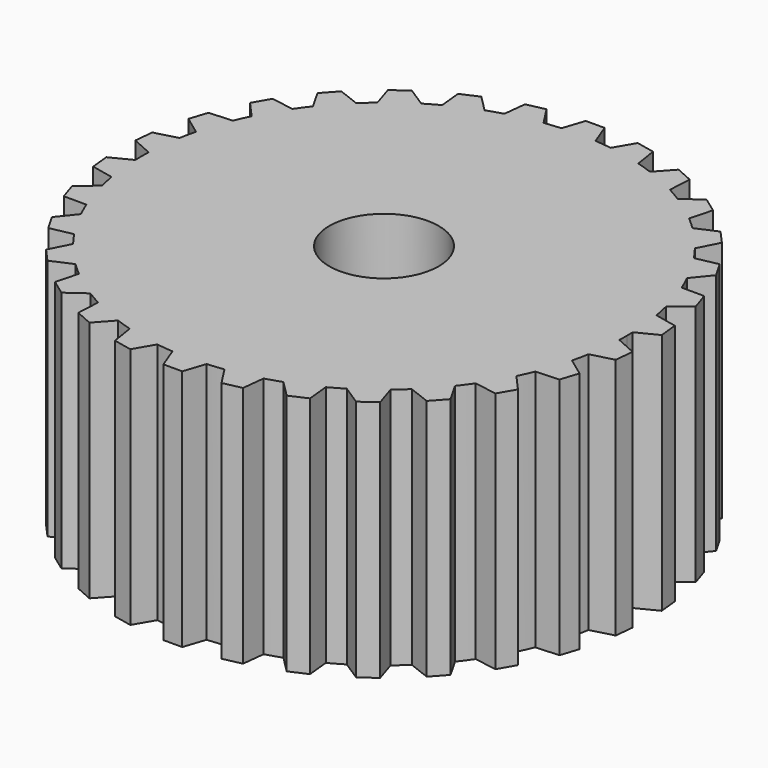
from build123d import *

# Parameters (mm, degrees)
F1_DEPTH = 25
F2_R     = 5.6332582932
F3_DEPTH = 25.001


with BuildPart() as f1:
    # F0 (on Top) → F1 (new body)
    with BuildSketch(Plane.XY):
        with BuildLine():
            ThreePointArc((24.9826599942, -0.9309670328), (24.9956646226, -0.4655642523), (25, 0))
            ThreePointArc((25, 0), (24.9969712413, 0.3891384843), (24.9878856992, 0.77818268))
            ThreePointArc((24.9878856992, 0.77818268), (24.8709209984, 2.5371812491), (24.6302878631, 4.283563911))
            ThreePointArc((24.6302878631, 4.283563911), (24.4694678339, 5.1230014568), (24.2800471673, 5.956451087))
            ThreePointArc((24.2800471673, 5.956451087), (23.7999220592, 7.6526929884), (23.2014539632, 9.3108825571))
            ThreePointArc((23.2014539632, 9.3108825571), (22.869619358, 10.0985400143), (22.5110540656, 10.8743939994))
            ThreePointArc((22.5110540656, 10.8743939994), (21.6887523213, 12.4337453224), (20.7586051922, 13.9312709568))
            ThreePointArc((20.7586051922, 13.9312709568), (20.2702587756, 14.6327239149), (19.7582198813, 15.3170737128))
            ThreePointArc((19.7582198813, 15.3170737128), (18.6296800329, 16.6713833221), (17.4085057635, 17.9427959661))
            ThreePointArc((17.4085057635, 17.9427959661), (16.7849906172, 18.5273875649), (16.1418566776, 19.0903238055))
            ThreePointArc((16.1418566776, 19.0903238055), (14.7564013318, 20.1804018725), (13.2975710976, 21.1701346926))
            ThreePointArc((13.2975710976, 21.1701346926), (12.5661378255, 21.6123154741), (11.82001688, 22.0292351424))
            ThreePointArc((11.82001688, 22.0292351424), (10.2381970835, 22.8074400247), (8.6054687659, 23.4722369475))
            ThreePointArc((8.6054687659, 23.4722369475), (7.7980845118, 23.7526814896), (6.9815856259, 24.0053631955))
            ThreePointArc((6.9815856259, 24.0053631955), (5.2725344943, 24.4376836056), (3.5372661556, 24.7484898154))
            ThreePointArc((3.5372661556, 24.7484898154), (2.6892174855, 24.854941346), (1.8380255786, 24.9323416865))
            ThreePointArc((1.8380255786, 24.9323416865), (0.9196352096, 24.9830796957), (0, 25))
            ThreePointArc((0, 25), (-0.8432457973, 24.9857746833), (-1.6855319595, 24.943114922))
            ThreePointArc((-1.6855319595, 24.943114922), (-2.5371812491, 24.8709209984), (-3.3858650063, 24.7696572071))
            ThreePointArc((-3.3858650063, 24.7696572071), (-5.1230014568, 24.4694678339), (-6.8346642398, 24.0476062162))
            ThreePointArc((-6.8346642398, 24.0476062162), (-7.6526929884, 23.7999220592), (-8.4617770432, 23.5244198498))
            ThreePointArc((-8.4617770432, 23.5244198498), (-10.0985400143, 22.869619358), (-11.6850888965, 22.1011017255))
            ThreePointArc((-11.6850888965, 22.1011017255), (-12.4337453224, 21.6887523213), (-13.1678688193, 21.2510524624))
            ThreePointArc((-13.1678688193, 21.2510524624), (-14.6327239149, 20.2702587756), (-16.0248190972, 19.1886730365))
            ThreePointArc((-16.0248190972, 19.1886730365), (-16.6713833221, 18.6296800329), (-17.2984615414, 18.0489121085))
            ThreePointArc((-17.2984615414, 18.0489121085), (-18.5273875649, 16.7849906172), (-19.6641878077, 15.4376072584))
            ThreePointArc((-19.6641878077, 15.4376072584), (-20.1804018725, 14.7564013318), (-20.673028487, 14.0579476871))
            ThreePointArc((-20.673028487, 14.0579476871), (-21.6123154741, 12.5661378255), (-22.4441371517, 11.0118439652))
            ThreePointArc((-22.4441371517, 11.0118439652), (-22.8074400247, 10.2381970835), (-23.1440848876, 9.4525834943))
            ThreePointArc((-23.1440848876, 9.4525834943), (-23.7526814896, 7.7980845118), (-24.2431700033, 6.1048102501))
            ThreePointArc((-24.2431700033, 6.1048102501), (-24.4376836056, 5.2725344943), (-24.6036337208, 4.4340960443))
            ThreePointArc((-24.6036337208, 4.4340960443), (-24.854941346, 2.6892174855), (-24.9826599942, 0.9309670328))
            ThreePointArc((-24.9826599942, 0.9309670328), (-24.9998831479, 0.0764368473), (-24.9878856992, -0.77818268))
            ThreePointArc((-24.9878856992, -0.77818268), (-24.8709209984, -2.5371812491), (-24.6302878631, -4.283563911))
            ThreePointArc((-24.6302878631, -4.283563911), (-24.4694678339, -5.1230014568), (-24.2800471673, -5.956451087))
            ThreePointArc((-24.2800471673, -5.956451087), (-23.7999220592, -7.6526929884), (-23.2014539632, -9.3108825571))
            ThreePointArc((-23.2014539632, -9.3108825571), (-22.869619358, -10.0985400143), (-22.5110540656, -10.8743939994))
            ThreePointArc((-22.5110540656, -10.8743939994), (-21.6887523213, -12.4337453224), (-20.7586051922, -13.9312709568))
            ThreePointArc((-20.7586051922, -13.9312709568), (-20.2702587756, -14.6327239149), (-19.7582198813, -15.3170737128))
            ThreePointArc((-19.7582198813, -15.3170737128), (-18.6296800329, -16.6713833221), (-17.4085057635, -17.9427959661))
            ThreePointArc((-17.4085057635, -17.9427959661), (-16.7849906172, -18.5273875649), (-16.1418566776, -19.0903238055))
            ThreePointArc((-16.1418566776, -19.0903238055), (-14.7564013318, -20.1804018725), (-13.2975710976, -21.1701346926))
            ThreePointArc((-13.2975710976, -21.1701346926), (-12.5661378255, -21.6123154741), (-11.82001688, -22.0292351424))
            ThreePointArc((-11.82001688, -22.0292351424), (-10.2381970835, -22.8074400247), (-8.6054687659, -23.4722369475))
            ThreePointArc((-8.6054687659, -23.4722369475), (-7.7980845118, -23.7526814896), (-6.9815856259, -24.0053631955))
            ThreePointArc((-6.9815856259, -24.0053631955), (-5.2725344943, -24.4376836056), (-3.5372661556, -24.7484898154))
            ThreePointArc((-3.5372661556, -24.7484898154), (-2.6892174855, -24.854941346), (-1.8380255786, -24.9323416865))
            ThreePointArc((-1.8380255786, -24.9323416865), (-0.0764368473, -24.9998831479), (1.6855319595, -24.943114922))
            ThreePointArc((1.6855319595, -24.943114922), (2.5371812491, -24.8709209984), (3.3858650063, -24.7696572071))
            ThreePointArc((3.3858650063, -24.7696572071), (5.1230014568, -24.4694678339), (6.8346642398, -24.0476062162))
            ThreePointArc((6.8346642398, -24.0476062162), (7.6526929884, -23.7999220592), (8.4617770432, -23.5244198498))
            ThreePointArc((8.4617770432, -23.5244198498), (10.0985400143, -22.869619358), (11.6850888965, -22.1011017255))
            ThreePointArc((11.6850888965, -22.1011017255), (12.4337453224, -21.6887523213), (13.1678688193, -21.2510524624))
            ThreePointArc((13.1678688193, -21.2510524624), (14.6327239149, -20.2702587756), (16.0248190972, -19.1886730365))
            ThreePointArc((16.0248190972, -19.1886730365), (16.6713833221, -18.6296800329), (17.2984615414, -18.0489121085))
            ThreePointArc((17.2984615414, -18.0489121085), (18.5273875649, -16.7849906172), (19.6641878077, -15.4376072584))
            ThreePointArc((19.6641878077, -15.4376072584), (20.1804018725, -14.7564013318), (20.673028487, -14.0579476871))
            ThreePointArc((20.673028487, -14.0579476871), (21.6123154741, -12.5661378255), (22.4441371517, -11.0118439652))
            ThreePointArc((22.4441371517, -11.0118439652), (22.8074400247, -10.2381970835), (23.1440848876, -9.4525834943))
            ThreePointArc((23.1440848876, -9.4525834943), (23.7526814896, -7.7980845118), (24.2431700033, -6.1048102501))
            ThreePointArc((24.2431700033, -6.1048102501), (24.4376836056, -5.2725344943), (24.6036337208, -4.4340960443))
            ThreePointArc((24.6036337208, -4.4340960443), (24.854941346, -2.6892174855), (24.9826599942, -0.9309670328))
        make_face()
        with BuildLine():
            ThreePointArc((24.6302878631, 4.283563911), (24.8709209984, 2.5371812491), (24.9878856992, 0.77818268))
            Line((24.9878856992, 0.77818268), (27.1162286769, 1.8601129156))
            Line((27.1162286769, 1.8601129156), (26.9136978769, 3.7870647602))
            Line((26.9136978769, 3.7870647602), (24.6302878631, 4.283563911))
        make_face()
        with BuildLine():
            Line((27.1129440427, -1.8913641228), (24.9826599942, -0.9309670328))
            ThreePointArc((24.9826599942, -0.9309670328), (24.854941346, -2.6892174855), (24.6036337208, -4.4340960443))
            Line((24.6036337208, -4.4340960443), (26.9104132427, -3.8183159673))
            Line((26.9104132427, -3.8183159673), (27.1129440427, -1.8913641228))
        make_face()
        with BuildLine():
            ThreePointArc((23.2014539632, 9.3108825571), (23.7999220592, 7.6526929884), (24.2800471673, 5.956451087))
            Line((24.2800471673, 5.956451087), (26.1369347999, 7.4572459383))
            Line((26.1369347999, 7.4572459383), (25.5381939676, 9.2999807407))
            Line((25.5381939676, 9.2999807407), (23.2014539632, 9.3108825571))
        make_face()
        with BuildLine():
            Line((26.1272244515, -7.4871313177), (24.2431700033, -6.1048102501))
            ThreePointArc((24.2431700033, -6.1048102501), (23.7526814896, -7.7980845118), (23.1440848876, -9.4525834943))
            Line((23.1440848876, -9.4525834943), (25.5284836192, -9.3298661202))
            Line((25.5284836192, -9.3298661202), (26.1272244515, -7.4871313177))
        make_face()
        with BuildLine():
            ThreePointArc((20.7586051922, 13.9312709568), (21.6887523213, 12.4337453224), (22.5110540656, 10.8743939994))
            Line((22.5110540656, 10.8743939994), (24.0153314531, 12.7284615297))
            Line((24.0153314531, 12.7284615297), (23.0465484361, 14.4064429367))
            Line((23.0465484361, 14.4064429367), (20.7586051922, 13.9312709568))
        make_face()
        with BuildLine():
            Line((23.9996197794, -12.7556749469), (22.4441371517, -11.0118439652))
            ThreePointArc((22.4441371517, -11.0118439652), (21.6123154741, -12.5661378255), (20.673028487, -14.0579476871))
            Line((20.673028487, -14.0579476871), (23.0308367624, -14.4336563539))
            Line((23.0308367624, -14.4336563539), (23.9996197794, -12.7556749469))
        make_face()
        with BuildLine():
            ThreePointArc((17.4085057635, 17.9427959661), (18.6296800329, 16.6713833221), (19.7582198813, 15.3170737128))
            Line((19.7582198813, 15.3170737128), (20.8441428836, 17.4433822743))
            Line((20.8441428836, 17.4433822743), (19.5476581484, 18.8832744465))
            Line((19.5476581484, 18.8832744465), (17.4085057635, 17.9427959661))
        make_face()
        with BuildLine():
            Line((20.82311656, -17.4667343724), (19.6641878077, -15.4376072584))
            ThreePointArc((19.6641878077, -15.4376072584), (18.5273875649, -16.7849906172), (17.2984615414, -18.0489121085))
            Line((17.2984615414, -18.0489121085), (19.5266318248, -18.9066265446))
            Line((19.5266318248, -18.9066265446), (20.82311656, -17.4667343724))
        make_face()
        with BuildLine():
            ThreePointArc((13.2975710976, 21.1701346926), (14.7564013318, 20.1804018725), (16.1418566776, 19.0903238055))
            Line((16.1418566776, 19.0903238055), (16.7619652487, 21.3959435108))
            Line((16.7619652487, 21.3959435108), (15.1944413994, 22.534816251))
            Line((15.1944413994, 22.534816251), (13.2975710976, 21.1701346926))
        make_face()
        with BuildLine():
            Line((16.7365432265, -21.4144136911), (16.0248190972, -19.1886730365))
            ThreePointArc((16.0248190972, -19.1886730365), (14.6327239149, -20.2702587756), (13.1678688193, -21.2510524624))
            Line((13.1678688193, -21.2510524624), (15.1690193773, -22.5532864312))
            Line((15.1690193773, -22.5532864312), (16.7365432265, -21.4144136911))
        make_face()
        with BuildLine():
            ThreePointArc((8.6054687659, 23.4722369475), (10.2381970835, 22.8074400247), (11.82001688, 22.0292351424))
            Line((11.82001688, 22.0292351424), (11.9472092996, 24.4133993468))
            Line((11.9472092996, 24.4133993468), (10.1771546504, 25.2014784512))
            Line((10.1771546504, 25.2014784512), (8.6054687659, 23.4722369475))
        make_face()
        with BuildLine():
            Line((11.9185026432, -24.4261803737), (11.6850888965, -22.1011017255))
            ThreePointArc((11.6850888965, -22.1011017255), (10.0985400143, -22.869619358), (8.4617770432, -23.5244198498))
            Line((8.4617770432, -23.5244198498), (10.148447994, -25.2142594781))
            Line((10.148447994, -25.2142594781), (11.9185026432, -24.4261803737))
        make_face()
        with BuildLine():
            ThreePointArc((3.5372661556, 24.7484898154), (5.2725344943, 24.4376836056), (6.9815856259, 24.0053631955))
            Line((6.9815856259, 24.0053631955), (6.6103029751, 26.3638724829))
            Line((6.6103029751, 26.3638724829), (4.7150774076, 26.7667151131))
            Line((4.7150774076, 26.7667151131), (3.5372661556, 24.7484898154))
        make_face()
        with BuildLine():
            Line((6.5795663031, -26.3704057642), (6.8346642398, -24.0476062162))
            ThreePointArc((6.8346642398, -24.0476062162), (5.1230014568, -24.4694678339), (3.3858650063, -24.7696572071))
            Line((3.3858650063, -24.7696572071), (4.6843407356, -26.7732483944))
            Line((4.6843407356, -26.7732483944), (6.5795663031, -26.3704057642))
        make_face()
        with BuildLine():
            ThreePointArc((0, 25), (0.9196352096, 24.9830796957), (1.8380255786, 24.9323416865))
            Line((1.8380255786, 24.9323416865), (0.9844946908, 27.1621178836))
            Line((0.9844946908, 27.1621178836), (-0.9530713432, 27.1621178836))
            Line((-0.9530713432, 27.1621178836), (-1.6855319595, 24.943114922))
            ThreePointArc((-1.6855319595, 24.943114922), (-0.8432457973, 24.9857746833), (0, 25))
        make_face()
        with BuildLine():
            Line((0.9530713432, -27.1621178836), (1.6855319595, -24.943114922))
            ThreePointArc((1.6855319595, -24.943114922), (-0.0764368473, -24.9998831479), (-1.8380255786, -24.9323416865))
            Line((-1.8380255786, -24.9323416865), (-0.9844946908, -27.1621178836))
            Line((-0.9844946908, -27.1621178836), (0.9530713432, -27.1621178836))
        make_face()
        with BuildLine():
            Line((-4.7150774076, -26.7667151131), (-3.5372661556, -24.7484898154))
            ThreePointArc((-3.5372661556, -24.7484898154), (-5.2725344943, -24.4376836056), (-6.9815856259, -24.0053631955))
            Line((-6.9815856259, -24.0053631955), (-6.6103029751, -26.3638724829))
            Line((-6.6103029751, -26.3638724829), (-4.7150774076, -26.7667151131))
        make_face()
        with BuildLine():
            ThreePointArc((-6.8346642398, 24.0476062162), (-5.1230014568, 24.4694678339), (-3.3858650063, 24.7696572071))
            Line((-3.3858650063, 24.7696572071), (-4.6843407356, 26.7732483944))
            Line((-4.6843407356, 26.7732483944), (-6.5795663031, 26.3704057642))
            Line((-6.5795663031, 26.3704057642), (-6.8346642398, 24.0476062162))
        make_face()
        with BuildLine():
            Line((-10.1771546504, -25.2014784512), (-8.6054687659, -23.4722369475))
            ThreePointArc((-8.6054687659, -23.4722369475), (-10.2381970835, -22.8074400247), (-11.82001688, -22.0292351424))
            Line((-11.82001688, -22.0292351424), (-11.9472092996, -24.4133993468))
            Line((-11.9472092996, -24.4133993468), (-10.1771546504, -25.2014784512))
        make_face()
        with BuildLine():
            ThreePointArc((-11.6850888965, 22.1011017255), (-10.0985400143, 22.869619358), (-8.4617770432, 23.5244198498))
            Line((-8.4617770432, 23.5244198498), (-10.148447994, 25.2142594781))
            Line((-10.148447994, 25.2142594781), (-11.9185026432, 24.4261803737))
            Line((-11.9185026432, 24.4261803737), (-11.6850888965, 22.1011017255))
        make_face()
        with BuildLine():
            Line((-15.1944413994, -22.534816251), (-13.2975710976, -21.1701346926))
            ThreePointArc((-13.2975710976, -21.1701346926), (-14.7564013318, -20.1804018725), (-16.1418566776, -19.0903238055))
            Line((-16.1418566776, -19.0903238055), (-16.7619652487, -21.3959435108))
            Line((-16.7619652487, -21.3959435108), (-15.1944413994, -22.534816251))
        make_face()
        with BuildLine():
            ThreePointArc((-16.0248190972, 19.1886730365), (-14.6327239149, 20.2702587756), (-13.1678688193, 21.2510524624))
            Line((-13.1678688193, 21.2510524624), (-15.1690193773, 22.5532864312))
            Line((-15.1690193773, 22.5532864312), (-16.7365432265, 21.4144136911))
            Line((-16.7365432265, 21.4144136911), (-16.0248190972, 19.1886730365))
        make_face()
        with BuildLine():
            Line((-19.5476581484, -18.8832744465), (-17.4085057635, -17.9427959661))
            ThreePointArc((-17.4085057635, -17.9427959661), (-18.6296800329, -16.6713833221), (-19.7582198813, -15.3170737128))
            Line((-19.7582198813, -15.3170737128), (-20.8441428836, -17.4433822743))
            Line((-20.8441428836, -17.4433822743), (-19.5476581484, -18.8832744465))
        make_face()
        with BuildLine():
            ThreePointArc((-19.6641878077, 15.4376072584), (-18.5273875649, 16.7849906172), (-17.2984615414, 18.0489121085))
            Line((-17.2984615414, 18.0489121085), (-19.5266318248, 18.9066265446))
            Line((-19.5266318248, 18.9066265446), (-20.82311656, 17.4667343724))
            Line((-20.82311656, 17.4667343724), (-19.6641878077, 15.4376072584))
        make_face()
        with BuildLine():
            Line((-23.0465484361, -14.4064429367), (-20.7586051922, -13.9312709568))
            ThreePointArc((-20.7586051922, -13.9312709568), (-21.6887523213, -12.4337453224), (-22.5110540656, -10.8743939994))
            Line((-22.5110540656, -10.8743939994), (-24.0153314531, -12.7284615297))
            Line((-24.0153314531, -12.7284615297), (-23.0465484361, -14.4064429367))
        make_face()
        with BuildLine():
            ThreePointArc((-22.4441371517, 11.0118439652), (-21.6123154741, 12.5661378255), (-20.673028487, 14.0579476871))
            Line((-20.673028487, 14.0579476871), (-23.0308367624, 14.4336563539))
            Line((-23.0308367624, 14.4336563539), (-23.9996197794, 12.7556749469))
            Line((-23.9996197794, 12.7556749469), (-22.4441371517, 11.0118439652))
        make_face()
        with BuildLine():
            Line((-25.5381939676, -9.2999807407), (-23.2014539632, -9.3108825571))
            ThreePointArc((-23.2014539632, -9.3108825571), (-23.7999220592, -7.6526929884), (-24.2800471673, -5.956451087))
            Line((-24.2800471673, -5.956451087), (-26.1369347999, -7.4572459383))
            Line((-26.1369347999, -7.4572459383), (-25.5381939676, -9.2999807407))
        make_face()
        with BuildLine():
            ThreePointArc((-24.2431700033, 6.1048102501), (-23.7526814896, 7.7980845118), (-23.1440848876, 9.4525834943))
            Line((-23.1440848876, 9.4525834943), (-25.5284836192, 9.3298661202))
            Line((-25.5284836192, 9.3298661202), (-26.1272244515, 7.4871313177))
            Line((-26.1272244515, 7.4871313177), (-24.2431700033, 6.1048102501))
        make_face()
        with BuildLine():
            Line((-26.9136978769, -3.7870647602), (-24.6302878631, -4.283563911))
            ThreePointArc((-24.6302878631, -4.283563911), (-24.8709209984, -2.5371812491), (-24.9878856992, -0.77818268))
            Line((-24.9878856992, -0.77818268), (-27.1162286769, -1.8601129156))
            Line((-27.1162286769, -1.8601129156), (-26.9136978769, -3.7870647602))
        make_face()
        with BuildLine():
            ThreePointArc((-24.9826599942, 0.9309670328), (-24.854941346, 2.6892174855), (-24.6036337208, 4.4340960443))
            Line((-24.6036337208, 4.4340960443), (-26.9104132427, 3.8183159673))
            Line((-26.9104132427, 3.8183159673), (-27.1129440427, 1.8913641228))
            Line((-27.1129440427, 1.8913641228), (-24.9826599942, 0.9309670328))
        make_face()
    extrude(amount=F1_DEPTH)

    # F2 (on face) → F3 (cut, through all)
    with BuildSketch(Plane(origin=(0, 0, 0), x_dir=(1, 0, 0), z_dir=(0, 0, -1))):
        Circle(F2_R)
    extrude(amount=-F3_DEPTH, mode=Mode.SUBTRACT)


solid = f1.part
